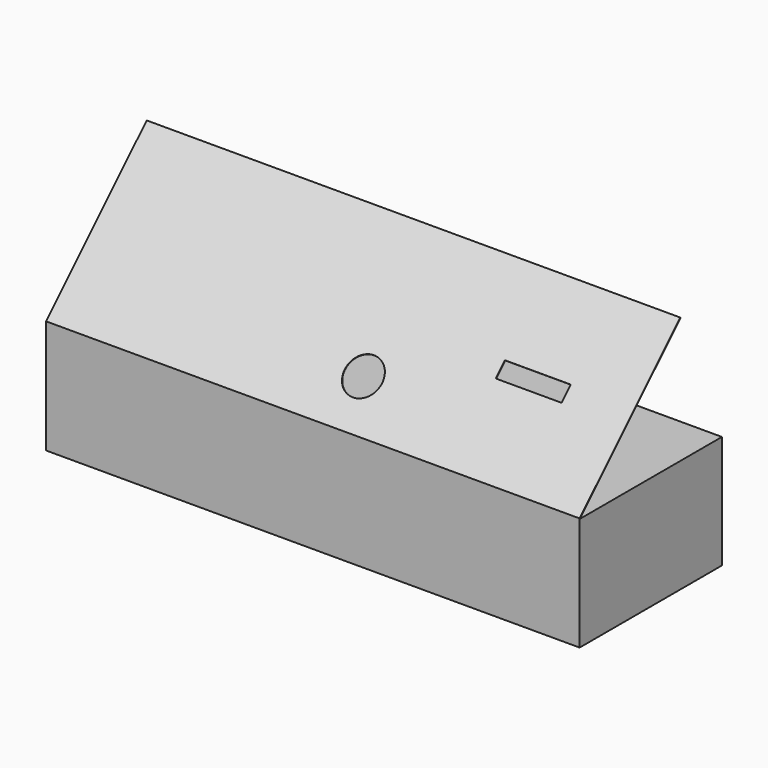
from build123d import *

# Parameters (mm, degrees)
F1_DEPTH = 209.55
F2_W     = 51.59375
F2_H     = 12.7
F3_DEPTH = 0.4064


# Not quite as in the source:
# - the dataset's text gives a spline's control points without its knots; the knots are read off the source's solid


with BuildPart() as f1:
    # F0 (on Right) → F1 (new body, symmetric)
    with BuildSketch(Plane.YZ):
        Polygon((-139.7, 0), (0, 0), (0, 88.9), (-139.2936, 88.9), (-139.2936, 89.154), (-40.6298144724, 187.8177855276), (-40.9171826682, 188.1051537235), (-139.7, 89.3223363917), align=None)
    extrude(amount=F1_DEPTH, both=True)

    # F2 (on face) → F3 (cut, through all)
    with BuildSketch(Plane(origin=(0, -114.5111681959, 114.5111681959), x_dir=(1, 0, 0), z_dir=(0, -0.7071067812, 0.7071067812))):
        with Locations((133.3471488731, 34.6446699547)):
            Rectangle(F2_W, F2_H)
        with BuildLine():
            add(Edge.make_bspline(
                [(29.4310752731, 11.2932815547), (26.7125386731, 14.0114625547), (22.8919722731, 15.5939587547), (19.0471996731, 15.5939587547)],
                knots=[7, 7, 7, 7, 8, 8, 8, 8], degree=3))
            add(Edge.make_bspline(
                [(19.0471996731, 15.5939587547), (15.2031636731, 15.5939587547), (11.3825972731, 14.0114625547), (8.6636796731, 11.2932815547)],
                knots=[0, 0, 0, 0, 1, 1, 1, 1], degree=3))
            add(Edge.make_bspline(
                [(8.6636796731, 11.2932815547), (5.9454986731, 8.5747703547), (4.3628246731, 4.7539753547), (4.3628246731, 0.9095837547), (4.3628246731, -2.9346046453), (5.9454986731, -6.7553996453), (8.6636796731, -9.4735806453)],
                knots=[1, 1, 1, 1, 2, 2, 2, 3, 3, 3, 3], degree=3))
            add(Edge.make_bspline(
                [(8.6636796731, -9.4735806453), (11.3825972731, -12.1920918453), (15.2031636731, -13.7747912453), (19.0471996731, -13.7747912453), (22.8919722731, -13.7747912453), (26.7125386731, -12.1920918453), (29.4310752731, -9.4735806453), (32.1492816731, -6.7553996453), (33.7315746731, -2.9346046453), (33.7315746731, 0.9095837547), (33.7315746731, 4.7539753547), (32.1492816731, 8.5747703547), (29.4310752731, 11.2932815547)],
                knots=[3, 3, 3, 3, 4, 4, 4, 5, 5, 5, 6, 6, 6, 7, 7, 7, 7], degree=3))
        make_face()
    extrude(amount=-F3_DEPTH, mode=Mode.SUBTRACT)


solid = f1.part
